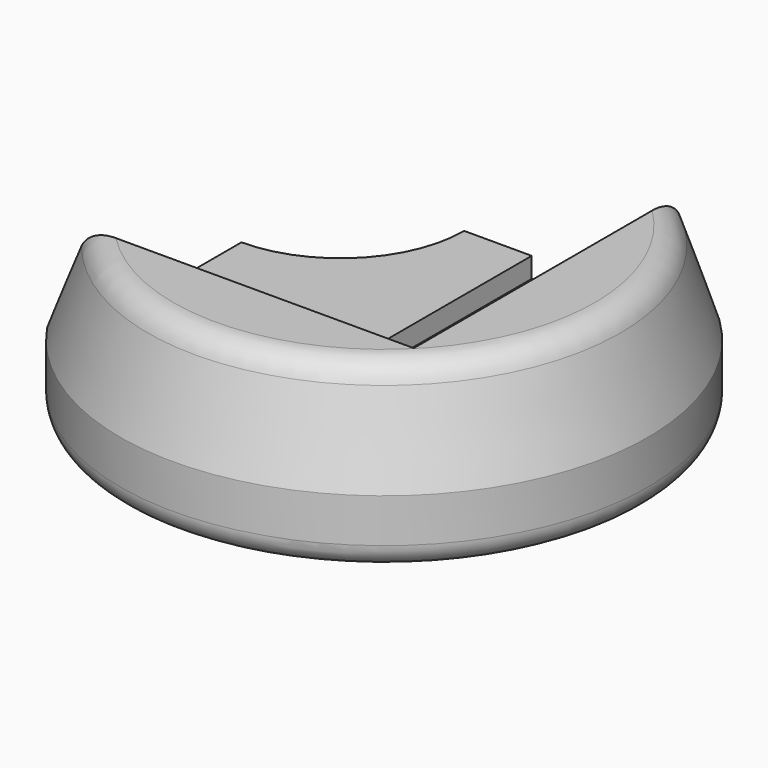
from build123d import *

# Parameters (mm, degrees)
F1_DEPTH = 6.5
F2_DEPTH = 3.5
F3_DEPTH = 25
F4_R     = 3.49999
F5_SIZE2 = 15
F5_SIZE  = 5
F6_R     = 4


# Not quite as in the source:
# - a fillet or chamfer is up to 0.001 mm smaller than in the source, because OpenCascade refuses the exact size


with BuildPart() as f1:
    # F0 (on Top) → F1 (new body)
    with BuildSketch(Plane.XY):
        with BuildLine():
            Line((-1.6568542495, 1.6568542495), (-1.6568542495, 30))
            Line((-1.6568542495, 30), (-11.6568542495, 30))
            ThreePointArc((-11.6568542495, 30), (-17.0460019087, 17.0460019087), (-30, 11.6568542495))
            Line((-30, 11.6568542495), (-30, 1.6568542495))
            Line((-30, 1.6568542495), (-1.6568542495, 1.6568542495))
        make_face()
    extrude(amount=F1_DEPTH)

    # F0 (on Top) → F2 (join)
    with BuildSketch(Plane.XY):
        Polygon((24.3431457505, -24.3431457505), (24.3431457505, 30), (-1.6568542495, 30), (-1.6568542495, 1.6568542495), (-30, 1.6568542495), (-30, -24.3431457505), align=None)
    extrude(amount=F2_DEPTH)

    # F0 (on Top) → F3 (join)
    with BuildSketch(Plane.XY):
        with BuildLine():
            ThreePointArc((-30, -24.3431457505), (30, -30), (24.3431457505, 30))
            Line((24.3431457505, 30), (24.3431457505, -24.3431457505))
            Line((24.3431457505, -24.3431457505), (-30, -24.3431457505))
        make_face()
    extrude(amount=F3_DEPTH)

    # F4 (radius 3.5 in the source; OpenCascade refuses exactly that, so slightly less here)
    f4_edges = [f1.edges().sort_by_distance(p)[0] for p in [
        (30, -30, 0),
        (-30, -6.343146, 0),
        (6.343146, 30, 0),
    ]]
    fillet(f4_edges, radius=F4_R)

    # F5
    f5_edges = [f1.edges().sort_by_distance(p)[0] for p in [
        (30, -30, 25),
    ]]
    f5_side = f1.faces().sort_by_distance((29.285433, -29.285433, 25))[0]
    chamfer(f5_edges, length=F5_SIZE, length2=F5_SIZE2, reference=f5_side)

    # F6
    f6_edges = [f1.edges().sort_by_distance(p)[0] for p in [
        (26.464466, -26.464466, 25),
    ]]
    fillet(f6_edges, radius=F6_R)


solid = f1.part
